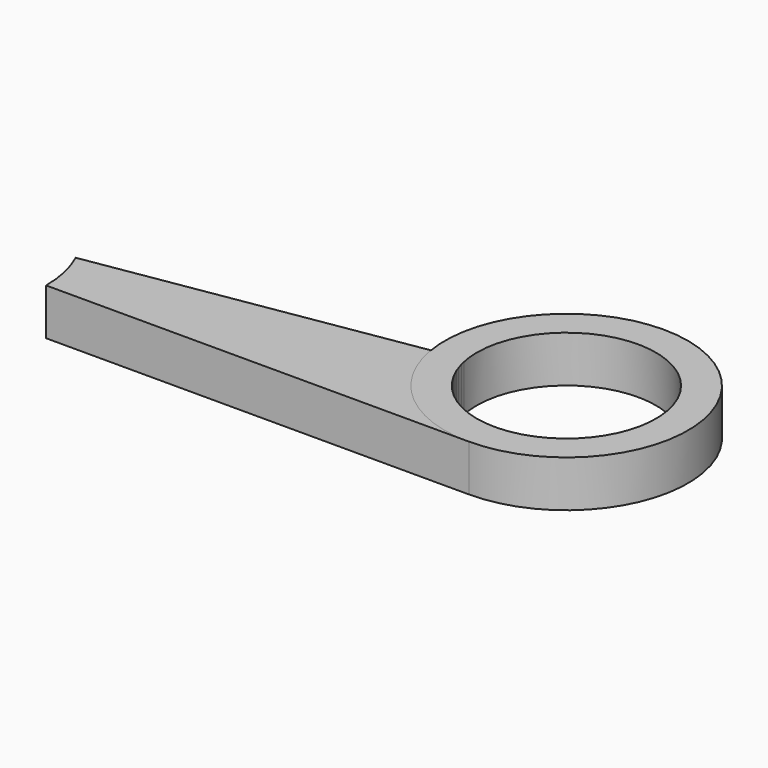
from build123d import *

# Parameters (mm, degrees)
F0_W          = 77.2340670228
F0_H          = 17.2310173512
F1_DEPTH      = 6.596820429
F1_FACE_W     = 77.2340670228
F1_FACE_H     = 6.596820429
F2_ANGLE_BACK = 9.2222213089
F2_ANGLE      = 18.4444426177
F1_FACE1_W    = 17.2310173512
F1_FACE1_H    = 6.596820429
F5_D          = 25.4
F5_2_D        = 25.4
F1_FACE2_W    = 17.2310173512
F1_FACE2_H    = 6.596820429


# Not quite as in the source:
# - the program builds the solid bodies; features that only make, move or delete a surface that nothing else refers to are left out


with BuildPart() as f1:
    # F0 (on Top) → F1 (new body)
    with BuildSketch(Plane.XY):
        with Locations((-38.6170335114, -8.6155086756)):
            Rectangle(F0_W, F0_H)
    extrude(amount=F1_DEPTH)

    # F1_face (on face) → F2 (revolve, cut)
    with BuildSketch(Plane(origin=(-38.6170335114, 0, 3.2984102145), x_dir=(-1, 0, 0), z_dir=(0, 1, 0)), mode=Mode.PRIVATE) as f2_sk:
        Rectangle(F1_FACE_W, F1_FACE_H)
    revolve(f2_sk.sketch.rotate(Axis((0, 0, 3.2984102145), (0, 0, -1)), -F2_ANGLE_BACK), axis=Axis((0, 0, 3.2984102145), (0, 0, -1)), revolution_arc=F2_ANGLE, mode=Mode.SUBTRACT)

    # F5 (through all)
    with Locations(Plane.XY.offset(6.596820429)):
        with Locations((0, 0)):
            Hole(F5_D / 2)

    # F1_face2 (on face) → F6 (revolve, cut)
    with BuildSketch(Plane(origin=(-77.2340670228, -8.6155086756, 3.2984102145), x_dir=(0, -1, 0), z_dir=(-1, 0, 0))):
        Rectangle(F1_FACE2_W, F1_FACE2_H)
    revolve(axis=Axis((-77.2340670228, -17.2310173512, 3.2984102145), (0, 0, -1)), mode=Mode.SUBTRACT)


with BuildPart() as f3:
    # F1_face1 (on face) → F3 (revolve)
    with BuildSketch(Plane(origin=(0, -8.6155086756, 3.2984102145), x_dir=(0, 1, 0), z_dir=(1, 0, 0))):
        Rectangle(F1_FACE1_W, F1_FACE1_H)
    revolve(axis=Axis((0, 0, 3.2984102145), (0, 0, -1)))

    # F5#2 (through all)
    with Locations(Plane.XY.offset(6.596820429)):
        with Locations((0, 0)):
            Hole(F5_2_D / 2)


solid = Compound([f1.part, f3.part])
